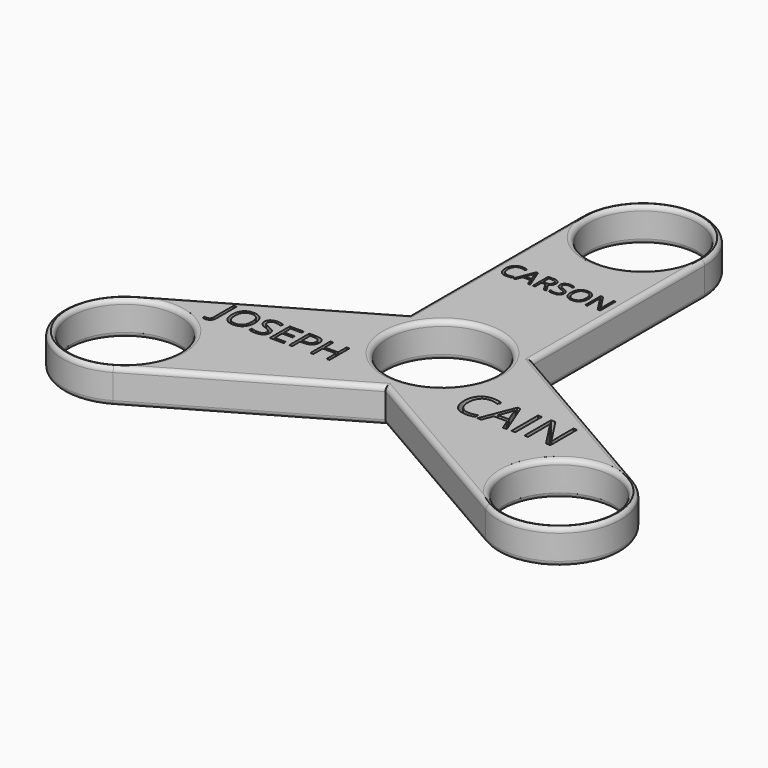
from build123d import *

# Parameters (mm, degrees)
F2_DEPTH      = 7
F1_R          = 11
F1_R_2        = 11.1
F3_DEPTH      = 25.4
F4_T8_DEPTH   = 46.0831216351
F4_T13_DEPTH  = 46.0831216351
F4_T18_DEPTH  = 46.0831216351
F4_T23_DEPTH  = 46.0831216351
F4_T28_DEPTH  = 46.0831216351
F4_T37_DEPTH  = 46.0831216351
F4_T42_DEPTH  = 46.0831216351
F4_T51_DEPTH  = 46.0831216351
F4_T56_DEPTH  = 46.0831216351
F4_T59_ANGLE  = 180
F4_T61_ANGLE  = 180
F4_T63_ANGLE  = 180
F4_T67_DEPTH  = 46.0831216351
F4_T70_ANGLE  = 180
F4_T74_DEPTH  = 46.0831216351
F4_T77_ANGLE  = 180
F4_T81_DEPTH  = 46.0831216351
F4_T84_ANGLE  = 180
F4_T89_DEPTH  = 46.0831216351
F4_T93_DEPTH  = 46.0831216351
F4_T100_DEPTH = 46.0831216351
F4_T104_DEPTH = 46.0831216351
F4_T111_DEPTH = 46.0831216351
F4_T115_DEPTH = 46.0831216351
F4_T122_DEPTH = 46.0831216351
F4_T126_DEPTH = 46.0831216351
F4_T133_DEPTH = 46.0831216351
F4_T137_DEPTH = 46.0831216351
F4_T144_DEPTH = 46.0831216351
F4_T148_DEPTH = 46.0831216351
F5_R          = 1
F6_TEXT_SIZE  = 5.4523334279
F7_DEPTH      = 3
F8_TEXT_SIZE  = 7.1097765769
F9_DEPTH      = 3
F10_TEXT_SIZE = 9.4424461066
F11_DEPTH     = 3


# Not quite as in the source:
# - a fillet or chamfer that OpenCascade refuses, or shapes differently, is made with other operations: its cross-section is extruded or revolved along the edge and cut away or added
# - Text() gives the source's letters only with a copy of the font that has no kerning and outlines rounded to 1/6400 em; it was checked with that copy


with BuildPart() as f2:
    # F0 (on Top) → F2 (new body)
    with BuildSketch(Plane.XY):
        with BuildLine():
            ThreePointArc((12.5, 50.8), (0, 63.3), (-12.5, 50.8))
            Line((-12.5, 50.8), (-12.5, 7.2168783649))
            Line((-12.5, 7.2168783649), (-50.2440905122, -14.5746824527))
            ThreePointArc((-50.2440905122, -14.5746824527), (-54.8194080596, -31.65), (-37.7440905122, -36.2253175473))
            Line((-37.7440905122, -36.2253175473), (0, -14.4337567297))
            Line((0, -14.4337567297), (37.7440905122, -36.2253175473))
            ThreePointArc((37.7440905122, -36.2253175473), (54.8194080596, -31.65), (50.2440905122, -14.5746824527))
            Line((50.2440905122, -14.5746824527), (12.5, 7.2168783649))
            Line((12.5, 7.2168783649), (12.5, 50.8))
        make_face()
    extrude(amount=F2_DEPTH)

    # F1 (on Top) → F3 (cut)
    with BuildSketch(Plane.XY):
        with Locations((0, 50.8)):
            Circle(F1_R)
        with Locations((-43.9940905122, -25.4)):
            Circle(F1_R)
        with Locations((43.9940905122, -25.4)):
            Circle(F1_R)
        Circle(F1_R_2)
    extrude(amount=F3_DEPTH, mode=Mode.SUBTRACT)

    # F4: fillet of radius 1 on 15 edges, made by hand

    # F4_s1 → F4_t2 (revolve, cut)
    with BuildSketch(Plane.XZ.offset(-50.8)):
        with BuildLine():
            ThreePointArc((12, 7), (11.2928932188, 6.7071067812), (11, 6))
            Line((11, 6), (11, 7))
            Line((11, 7), (12, 7))
        make_face()
    revolve(axis=Axis((0, 50.8, 7), (0, 0, -1)), mode=Mode.SUBTRACT)

    # F4_s3 → F4_t4 (revolve, cut)
    with BuildSketch(Plane.XZ.offset(-50.8)):
        with BuildLine():
            ThreePointArc((12, 0), (11.2928932188, 0.2928932188), (11, 1))
            Line((11, 1), (11, 0))
            Line((11, 0), (12, 0))
        make_face()
    revolve(axis=Axis((0, 50.8, 0), (0, 0, 1)), mode=Mode.SUBTRACT)


with BuildPart() as f4_tool6:
    # F4_s7 → F4_t8 (new body)
    with BuildSketch(Plane.XZ.offset(-50.8)):
        with BuildLine():
            ThreePointArc((-11.5, 0), (-12.2071067812, 0.2928932188), (-12.5, 1))
            Line((-12.5, 1), (-12.5, 0))
            Line((-12.5, 0), (-11.5, 0))
        make_face()
    extrude(amount=F4_T8_DEPTH)

    split(bisect_by=Plane(origin=(-6.25, 10.8253175473, 0), x_dir=(0, 0, 1), z_dir=(-0.5, 0.8660254038, 0)), keep=Keep.TOP)


with BuildPart() as f2_1:
    add(f2.part)

    # F4_t5: cut F4_tool6
    add(f4_tool6.part, mode=Mode.SUBTRACT)


with BuildPart() as f4_tool11:
    # F4_s12 → F4_t13 (new body)
    with BuildSketch(Plane.XZ.offset(-4.7168783649)):
        with BuildLine():
            ThreePointArc((11.5, 0), (12.2071067812, 0.2928932188), (12.5, 1))
            Line((12.5, 1), (12.5, 0))
            Line((12.5, 0), (11.5, 0))
        make_face()
    extrude(amount=-F4_T13_DEPTH)

    split(bisect_by=Plane(origin=(6.25, 10.8253175473, 0), x_dir=(0, 0, 1), z_dir=(0.5, 0.8660254038, 0)), keep=Keep.TOP)


with BuildPart() as f2_2:
    add(f2_1.part)

    # F4_t10: cut F4_tool11
    add(f4_tool11.part, mode=Mode.SUBTRACT)


with BuildPart() as f4_tool16:
    # F4_s17 → F4_t18 (new body)
    with BuildSketch(Plane.XZ.offset(-4.7168783649)):
        with BuildLine():
            ThreePointArc((11.5, 7), (12.2071067812, 6.7071067812), (12.5, 6))
            Line((12.5, 6), (12.5, 7))
            Line((12.5, 7), (11.5, 7))
        make_face()
    extrude(amount=-F4_T18_DEPTH)

    split(bisect_by=Plane(origin=(6.25, 10.8253175473, 0), x_dir=(0, 0, 1), z_dir=(0.5, 0.8660254038, 0)), keep=Keep.TOP)


with BuildPart() as f2_3:
    add(f2_2.part)

    # F4_t15: cut F4_tool16
    add(f4_tool16.part, mode=Mode.SUBTRACT)


with BuildPart() as f4_tool21:
    # F4_s22 → F4_t23 (new body)
    with BuildSketch(Plane(origin=(-4.0849364905, -2.3584391824, 0), x_dir=(0, 0, 1), z_dir=(-0.8660254038, -0.5, 0))):
        with BuildLine():
            ThreePointArc((0, 11.5), (0.2928932188, 12.2071067812), (1, 12.5))
            Line((1, 12.5), (0, 12.5))
            Line((0, 12.5), (0, 11.5))
        make_face()
    extrude(amount=F4_T23_DEPTH)

    split(bisect_by=Plane.YZ.offset(-12.5), keep=Keep.BOTTOM)


with BuildPart() as f2_4:
    add(f2_3.part)

    # F4_t20: cut F4_tool21
    add(f4_tool21.part, mode=Mode.SUBTRACT)


with BuildPart() as f4_tool26:
    # F4_s27 → F4_t28 (new body)
    with BuildSketch(Plane(origin=(-4.0849364905, -2.3584391824, 0), x_dir=(0, 0, 1), z_dir=(-0.8660254038, -0.5, 0))):
        with BuildLine():
            ThreePointArc((7, 11.5), (6.7071067812, 12.2071067812), (6, 12.5))
            Line((6, 12.5), (7, 12.5))
            Line((7, 12.5), (7, 11.5))
        make_face()
    extrude(amount=F4_T28_DEPTH)

    split(bisect_by=Plane.YZ.offset(-12.5), keep=Keep.BOTTOM)


with BuildPart() as f2_5:
    add(f2_4.part)

    # F4_t25: cut F4_tool26
    add(f4_tool26.part, mode=Mode.SUBTRACT)

    # F4_s30 → F4_t31 (revolve, cut)
    with BuildSketch(Plane.XZ.offset(25.4)):
        with BuildLine():
            ThreePointArc((-31.9940905122, 0), (-32.7011972934, 0.2928932188), (-32.9940905122, 1))
            Line((-32.9940905122, 1), (-32.9940905122, 0))
            Line((-32.9940905122, 0), (-31.9940905122, 0))
        make_face()
    revolve(axis=Axis((-43.9940905122, -25.4, 0), (0, 0, 1)), mode=Mode.SUBTRACT)

    # F4_s32 → F4_t33 (revolve, cut)
    with BuildSketch(Plane.XZ.offset(25.4)):
        with BuildLine():
            ThreePointArc((-31.9940905122, 7), (-32.7011972934, 6.7071067812), (-32.9940905122, 6))
            Line((-32.9940905122, 6), (-32.9940905122, 7))
            Line((-32.9940905122, 7), (-31.9940905122, 7))
        make_face()
    revolve(axis=Axis((-43.9940905122, -25.4, 7), (0, 0, -1)), mode=Mode.SUBTRACT)


with BuildPart() as f4_tool35:
    # F4_s36 → F4_t37 (new body)
    with BuildSketch(Plane(origin=(43.9940905122, -25.4, 0), x_dir=(0, 0, 1), z_dir=(-0.8660254038, 0.5, 0))):
        with BuildLine():
            ThreePointArc((7, 11.5), (6.7071067812, 12.2071067812), (6, 12.5))
            Line((6, 12.5), (7, 12.5))
            Line((7, 12.5), (7, 11.5))
        make_face()
    extrude(amount=F4_T37_DEPTH)

    split(bisect_by=Plane.YZ.offset(12.5), keep=Keep.TOP)


with BuildPart() as f2_6:
    add(f2_5.part)

    # F4_t34: cut F4_tool35
    add(f4_tool35.part, mode=Mode.SUBTRACT)


with BuildPart() as f4_tool40:
    # F4_s41 → F4_t42 (new body)
    with BuildSketch(Plane(origin=(4.0849364905, -2.3584391824, 0), x_dir=(0, 0, 1), z_dir=(0.8660254038, -0.5, 0))):
        with BuildLine():
            ThreePointArc((6, 12.5), (6.7071067812, 12.2071067812), (7, 11.5))
            Line((7, 11.5), (7, 12.5))
            Line((7, 12.5), (6, 12.5))
        make_face()
    extrude(amount=F4_T42_DEPTH)

    split(bisect_by=Plane(origin=(6.25, -10.8253175473, 0), x_dir=(0, 0, 1), z_dir=(0.5, -0.8660254038, 0)), keep=Keep.TOP)


with BuildPart() as f2_7:
    add(f2_6.part)

    # F4_t39: cut F4_tool40
    add(f4_tool40.part, mode=Mode.SUBTRACT)

    # F4_s44 → F4_t45 (revolve, cut)
    with BuildSketch(Plane.XZ.offset(25.4)):
        with BuildLine():
            ThreePointArc((55.9940905122, 7), (55.2869837311, 6.7071067812), (54.9940905122, 6))
            Line((54.9940905122, 6), (54.9940905122, 7))
            Line((54.9940905122, 7), (55.9940905122, 7))
        make_face()
    revolve(axis=Axis((43.9940905122, -25.4, 7), (0, 0, -1)), mode=Mode.SUBTRACT)

    # F4_s46 → F4_t47 (revolve, cut)
    with BuildSketch(Plane.XZ.offset(25.4)):
        with BuildLine():
            ThreePointArc((55.9940905122, 0), (55.2869837311, 0.2928932188), (54.9940905122, 1))
            Line((54.9940905122, 1), (54.9940905122, 0))
            Line((54.9940905122, 0), (55.9940905122, 0))
        make_face()
    revolve(axis=Axis((43.9940905122, -25.4, 0), (0, 0, 1)), mode=Mode.SUBTRACT)


with BuildPart() as f4_tool49:
    # F4_s50 → F4_t51 (new body)
    with BuildSketch(Plane(origin=(4.0849364905, -2.3584391824, 0), x_dir=(0, 0, 1), z_dir=(0.8660254038, -0.5, 0))):
        with BuildLine():
            ThreePointArc((1, 12.5), (0.2928932188, 12.2071067812), (0, 11.5))
            Line((0, 11.5), (0, 12.5))
            Line((0, 12.5), (1, 12.5))
        make_face()
    extrude(amount=F4_T51_DEPTH)

    split(bisect_by=Plane(origin=(6.25, -10.8253175473, 0), x_dir=(0, 0, 1), z_dir=(0.5, -0.8660254038, 0)), keep=Keep.TOP)


with BuildPart() as f2_8:
    add(f2_7.part)

    # F4_t48: cut F4_tool49
    add(f4_tool49.part, mode=Mode.SUBTRACT)


with BuildPart() as f4_tool54:
    # F4_s55 → F4_t56 (new body)
    with BuildSketch(Plane(origin=(43.9940905122, -25.4, 0), x_dir=(0, 0, 1), z_dir=(-0.8660254038, 0.5, 0))):
        with BuildLine():
            ThreePointArc((0, 11.5), (0.2928932188, 12.2071067812), (1, 12.5))
            Line((1, 12.5), (0, 12.5))
            Line((0, 12.5), (0, 11.5))
        make_face()
    extrude(amount=F4_T56_DEPTH)

    split(bisect_by=Plane.YZ.offset(12.5), keep=Keep.TOP)


with BuildPart() as f2_9:
    add(f2_8.part)

    # F4_t53: cut F4_tool54
    add(f4_tool54.part, mode=Mode.SUBTRACT)

    # F4_s58 → F4_t59 (revolve, cut)
    with BuildSketch(Plane(origin=(43.9940905122, -25.4, 0), x_dir=(0, 0, 1), z_dir=(-0.8660254038, 0.5, 0))):
        with BuildLine():
            ThreePointArc((0, -11.5), (0.2928932188, -12.2071067812), (1, -12.5))
            Line((1, -12.5), (0, -12.5))
            Line((0, -12.5), (0, -11.5))
        make_face()
    revolve(axis=Axis((43.9940905122, -25.4, 0), (0, 0, 1)), revolution_arc=F4_T59_ANGLE, mode=Mode.SUBTRACT)

    # F4_s60 → F4_t61 (revolve, cut)
    with BuildSketch(Plane(origin=(43.9940905122, -25.4, 0), x_dir=(0, 0, 1), z_dir=(-0.8660254038, 0.5, 0))):
        with BuildLine():
            ThreePointArc((7, -11.5), (6.7071067812, -12.2071067812), (6, -12.5))
            Line((6, -12.5), (7, -12.5))
            Line((7, -12.5), (7, -11.5))
        make_face()
    revolve(axis=Axis((43.9940905122, -25.4, 7), (0, 0, 1)), revolution_arc=F4_T61_ANGLE, mode=Mode.SUBTRACT)

    # F4_s62 → F4_t63 (revolve, cut)
    with BuildSketch(Plane(origin=(-43.9940905122, -25.4, 0), x_dir=(0, 0, 1), z_dir=(0.8660254038, 0.5, 0))):
        with BuildLine():
            ThreePointArc((6, -12.5), (6.7071067812, -12.2071067812), (7, -11.5))
            Line((7, -11.5), (7, -12.5))
            Line((7, -12.5), (6, -12.5))
        make_face()
    revolve(axis=Axis((-43.9940905122, -25.4, 7), (0, 0, 1)), revolution_arc=F4_T63_ANGLE, mode=Mode.SUBTRACT)


with BuildPart() as f4_tool65:
    # F4_s66 → F4_t67 (new body)
    with BuildSketch(Plane(origin=(-43.9940905122, -25.4, 0), x_dir=(0, 0, 1), z_dir=(0.8660254038, 0.5, 0))):
        with BuildLine():
            ThreePointArc((6, 12.5), (6.7071067812, 12.2071067812), (7, 11.5))
            Line((7, 11.5), (7, 12.5))
            Line((7, 12.5), (6, 12.5))
        make_face()
    extrude(amount=F4_T67_DEPTH)

    split(bisect_by=Plane(origin=(-6.25, -10.8253175473, 0), x_dir=(0, 0, 1), z_dir=(-0.5, -0.8660254038, 0)), keep=Keep.TOP)


with BuildPart() as f2_10:
    add(f2_9.part)

    # F4_t64: cut F4_tool65
    add(f4_tool65.part, mode=Mode.SUBTRACT)

    # F4_s69 → F4_t70 (revolve, cut)
    with BuildSketch(Plane(origin=(-43.9940905122, -25.4, 0), x_dir=(0, 0, 1), z_dir=(0.8660254038, 0.5, 0))):
        with BuildLine():
            ThreePointArc((1, -12.5), (0.2928932188, -12.2071067812), (0, -11.5))
            Line((0, -11.5), (0, -12.5))
            Line((0, -12.5), (1, -12.5))
        make_face()
    revolve(axis=Axis((-43.9940905122, -25.4, 0), (0, 0, 1)), revolution_arc=F4_T70_ANGLE, mode=Mode.SUBTRACT)


with BuildPart() as f4_tool72:
    # F4_s73 → F4_t74 (new body)
    with BuildSketch(Plane(origin=(-43.9940905122, -25.4, 0), x_dir=(0, 0, 1), z_dir=(0.8660254038, 0.5, 0))):
        with BuildLine():
            ThreePointArc((1, 12.5), (0.2928932188, 12.2071067812), (0, 11.5))
            Line((0, 11.5), (0, 12.5))
            Line((0, 12.5), (1, 12.5))
        make_face()
    extrude(amount=F4_T74_DEPTH)

    split(bisect_by=Plane(origin=(-6.25, -10.8253175473, 0), x_dir=(0, 0, 1), z_dir=(-0.5, -0.8660254038, 0)), keep=Keep.TOP)


with BuildPart() as f2_11:
    add(f2_10.part)

    # F4_t71: cut F4_tool72
    add(f4_tool72.part, mode=Mode.SUBTRACT)

    # F4_s76 → F4_t77 (revolve, cut)
    with BuildSketch(Plane.XZ.offset(-50.8)):
        with BuildLine():
            ThreePointArc((11.5, 7), (12.2071067812, 6.7071067812), (12.5, 6))
            Line((12.5, 6), (12.5, 7))
            Line((12.5, 7), (11.5, 7))
        make_face()
    revolve(axis=Axis((0, 50.8, 7), (0, 0, 1)), revolution_arc=F4_T77_ANGLE, mode=Mode.SUBTRACT)


with BuildPart() as f4_tool79:
    # F4_s80 → F4_t81 (new body)
    with BuildSketch(Plane.XZ.offset(-50.8)):
        with BuildLine():
            ThreePointArc((-11.5, 7), (-12.2071067812, 6.7071067812), (-12.5, 6))
            Line((-12.5, 6), (-12.5, 7))
            Line((-12.5, 7), (-11.5, 7))
        make_face()
    extrude(amount=F4_T81_DEPTH)

    split(bisect_by=Plane(origin=(-6.25, 10.8253175473, 0), x_dir=(0, 0, 1), z_dir=(-0.5, 0.8660254038, 0)), keep=Keep.TOP)


with BuildPart() as f2_12:
    add(f2_11.part)

    # F4_t78: cut F4_tool79
    add(f4_tool79.part, mode=Mode.SUBTRACT)

    # F4_s83 → F4_t84 (revolve, cut)
    with BuildSketch(Plane.XZ.offset(-50.8)):
        with BuildLine():
            ThreePointArc((11.5, 0), (12.2071067812, 0.2928932188), (12.5, 1))
            Line((12.5, 1), (12.5, 0))
            Line((12.5, 0), (11.5, 0))
        make_face()
    revolve(axis=Axis((0, 50.8, 0), (0, 0, 1)), revolution_arc=F4_T84_ANGLE, mode=Mode.SUBTRACT)


with BuildPart() as f4_tool87:
    # F4_s88 → F4_t89 (new body)
    with BuildSketch(Plane(origin=(-4.0849364905, -2.3584391824, 0), x_dir=(0, 0, 1), z_dir=(-0.8660254038, -0.5, 0))):
        with BuildLine():
            ThreePointArc((0, 11.5), (0.2928932188, 12.2071067812), (1, 12.5))
            Line((1, 12.5), (0, 12.5))
            Line((0, 12.5), (0, 11.5))
        make_face()
    extrude(amount=F4_T89_DEPTH)

    split(bisect_by=Plane.YZ.offset(-12.5), keep=Keep.TOP)


with BuildPart() as f4_tool91:
    # F4_s92 → F4_t93 (new body)
    with BuildSketch(Plane.XZ.offset(-50.8)):
        with BuildLine():
            ThreePointArc((-11.5, 0), (-12.2071067812, 0.2928932188), (-12.5, 1))
            Line((-12.5, 1), (-12.5, 0))
            Line((-12.5, 0), (-11.5, 0))
        make_face()
    extrude(amount=F4_T93_DEPTH)

    split(bisect_by=Plane(origin=(-6.25, 10.8253175473, 0), x_dir=(0, 0, 1), z_dir=(0.5, -0.8660254038, 0)), keep=Keep.TOP)


with BuildPart() as f4_tool87_1:
    add(f4_tool87.part)

    # F4_t95: intersect F4_tool91
    add(f4_tool91.part, mode=Mode.INTERSECT)


with BuildPart() as f2_13:
    add(f2_12.part)

    # F4_t85: cut F4_tool87
    add(f4_tool87_1.part, mode=Mode.SUBTRACT)


with BuildPart() as f4_tool98:
    # F4_s99 → F4_t100 (new body)
    with BuildSketch(Plane(origin=(43.9940905122, -25.4, 0), x_dir=(0, 0, 1), z_dir=(-0.8660254038, 0.5, 0))):
        with BuildLine():
            ThreePointArc((0, 11.5), (0.2928932188, 12.2071067812), (1, 12.5))
            Line((1, 12.5), (0, 12.5))
            Line((0, 12.5), (0, 11.5))
        make_face()
    extrude(amount=F4_T100_DEPTH)

    split(bisect_by=Plane.YZ.offset(12.5), keep=Keep.BOTTOM)


with BuildPart() as f4_tool102:
    # F4_s103 → F4_t104 (new body)
    with BuildSketch(Plane.XZ.offset(-4.7168783649)):
        with BuildLine():
            ThreePointArc((11.5, 0), (12.2071067812, 0.2928932188), (12.5, 1))
            Line((12.5, 1), (12.5, 0))
            Line((12.5, 0), (11.5, 0))
        make_face()
    extrude(amount=-F4_T104_DEPTH)

    split(bisect_by=Plane(origin=(6.25, 10.8253175473, 0), x_dir=(0, 0, 1), z_dir=(-0.5, -0.8660254038, 0)), keep=Keep.TOP)


with BuildPart() as f4_tool98_1:
    add(f4_tool98.part)

    # F4_t106: intersect F4_tool102
    add(f4_tool102.part, mode=Mode.INTERSECT)


with BuildPart() as f2_14:
    add(f2_13.part)

    # F4_t96: cut F4_tool98
    add(f4_tool98_1.part, mode=Mode.SUBTRACT)


with BuildPart() as f4_tool109:
    # F4_s110 → F4_t111 (new body)
    with BuildSketch(Plane(origin=(43.9940905122, -25.4, 0), x_dir=(0, 0, 1), z_dir=(-0.8660254038, 0.5, 0))):
        with BuildLine():
            ThreePointArc((7, 11.5), (6.7071067812, 12.2071067812), (6, 12.5))
            Line((6, 12.5), (7, 12.5))
            Line((7, 12.5), (7, 11.5))
        make_face()
    extrude(amount=F4_T111_DEPTH)

    split(bisect_by=Plane.YZ.offset(12.5), keep=Keep.BOTTOM)


with BuildPart() as f4_tool113:
    # F4_s114 → F4_t115 (new body)
    with BuildSketch(Plane.XZ.offset(-4.7168783649)):
        with BuildLine():
            ThreePointArc((11.5, 7), (12.2071067812, 6.7071067812), (12.5, 6))
            Line((12.5, 6), (12.5, 7))
            Line((12.5, 7), (11.5, 7))
        make_face()
    extrude(amount=-F4_T115_DEPTH)

    split(bisect_by=Plane(origin=(6.25, 10.8253175473, 0), x_dir=(0, 0, 1), z_dir=(-0.5, -0.8660254038, 0)), keep=Keep.TOP)


with BuildPart() as f4_tool109_1:
    add(f4_tool109.part)

    # F4_t117: intersect F4_tool113
    add(f4_tool113.part, mode=Mode.INTERSECT)


with BuildPart() as f2_15:
    add(f2_14.part)

    # F4_t107: cut F4_tool109
    add(f4_tool109_1.part, mode=Mode.SUBTRACT)


with BuildPart() as f4_tool120:
    # F4_s121 → F4_t122 (new body)
    with BuildSketch(Plane(origin=(-4.0849364905, -2.3584391824, 0), x_dir=(0, 0, 1), z_dir=(-0.8660254038, -0.5, 0))):
        with BuildLine():
            ThreePointArc((7, 11.5), (6.7071067812, 12.2071067812), (6, 12.5))
            Line((6, 12.5), (7, 12.5))
            Line((7, 12.5), (7, 11.5))
        make_face()
    extrude(amount=F4_T122_DEPTH)

    split(bisect_by=Plane.YZ.offset(-12.5), keep=Keep.TOP)


with BuildPart() as f4_tool124:
    # F4_s125 → F4_t126 (new body)
    with BuildSketch(Plane.XZ.offset(-50.8)):
        with BuildLine():
            ThreePointArc((-11.5, 7), (-12.2071067812, 6.7071067812), (-12.5, 6))
            Line((-12.5, 6), (-12.5, 7))
            Line((-12.5, 7), (-11.5, 7))
        make_face()
    extrude(amount=F4_T126_DEPTH)

    split(bisect_by=Plane(origin=(-6.25, 10.8253175473, 0), x_dir=(0, 0, 1), z_dir=(0.5, -0.8660254038, 0)), keep=Keep.TOP)


with BuildPart() as f4_tool120_1:
    add(f4_tool120.part)

    # F4_t128: intersect F4_tool124
    add(f4_tool124.part, mode=Mode.INTERSECT)


with BuildPart() as f2_16:
    add(f2_15.part)

    # F4_t118: cut F4_tool120
    add(f4_tool120_1.part, mode=Mode.SUBTRACT)


with BuildPart() as f4_tool131:
    # F4_s132 → F4_t133 (new body)
    with BuildSketch(Plane(origin=(-43.9940905122, -25.4, 0), x_dir=(0, 0, 1), z_dir=(0.8660254038, 0.5, 0))):
        with BuildLine():
            ThreePointArc((6, 12.5), (6.7071067812, 12.2071067812), (7, 11.5))
            Line((7, 11.5), (7, 12.5))
            Line((7, 12.5), (6, 12.5))
        make_face()
    extrude(amount=F4_T133_DEPTH)

    split(bisect_by=Plane(origin=(-6.25, -10.8253175473, 0), x_dir=(0, 0, 1), z_dir=(0.5, 0.8660254038, 0)), keep=Keep.TOP)


with BuildPart() as f4_tool135:
    # F4_s136 → F4_t137 (new body)
    with BuildSketch(Plane(origin=(4.0849364905, -2.3584391824, 0), x_dir=(0, 0, 1), z_dir=(0.8660254038, -0.5, 0))):
        with BuildLine():
            ThreePointArc((6, 12.5), (6.7071067812, 12.2071067812), (7, 11.5))
            Line((7, 11.5), (7, 12.5))
            Line((7, 12.5), (6, 12.5))
        make_face()
    extrude(amount=F4_T137_DEPTH)

    split(bisect_by=Plane(origin=(6.25, -10.8253175473, 0), x_dir=(0, 0, 1), z_dir=(-0.5, 0.8660254038, 0)), keep=Keep.TOP)


with BuildPart() as f4_tool131_1:
    add(f4_tool131.part)

    # F4_t139: intersect F4_tool135
    add(f4_tool135.part, mode=Mode.INTERSECT)


with BuildPart() as f2_17:
    add(f2_16.part)

    # F4_t129: cut F4_tool131
    add(f4_tool131_1.part, mode=Mode.SUBTRACT)


with BuildPart() as f4_tool142:
    # F4_s143 → F4_t144 (new body)
    with BuildSketch(Plane(origin=(-43.9940905122, -25.4, 0), x_dir=(0, 0, 1), z_dir=(0.8660254038, 0.5, 0))):
        with BuildLine():
            ThreePointArc((1, 12.5), (0.2928932188, 12.2071067812), (0, 11.5))
            Line((0, 11.5), (0, 12.5))
            Line((0, 12.5), (1, 12.5))
        make_face()
    extrude(amount=F4_T144_DEPTH)

    split(bisect_by=Plane(origin=(-6.25, -10.8253175473, 0), x_dir=(0, 0, 1), z_dir=(0.5, 0.8660254038, 0)), keep=Keep.TOP)


with BuildPart() as f4_tool146:
    # F4_s147 → F4_t148 (new body)
    with BuildSketch(Plane(origin=(4.0849364905, -2.3584391824, 0), x_dir=(0, 0, 1), z_dir=(0.8660254038, -0.5, 0))):
        with BuildLine():
            ThreePointArc((1, 12.5), (0.2928932188, 12.2071067812), (0, 11.5))
            Line((0, 11.5), (0, 12.5))
            Line((0, 12.5), (1, 12.5))
        make_face()
    extrude(amount=F4_T148_DEPTH)

    split(bisect_by=Plane(origin=(6.25, -10.8253175473, 0), x_dir=(0, 0, 1), z_dir=(-0.5, 0.8660254038, 0)), keep=Keep.TOP)


with BuildPart() as f4_tool142_1:
    add(f4_tool142.part)

    # F4_t150: intersect F4_tool146
    add(f4_tool146.part, mode=Mode.INTERSECT)


with BuildPart() as f2_18:
    add(f2_17.part)

    # F4_t140: cut F4_tool142
    add(f4_tool142_1.part, mode=Mode.SUBTRACT)

    # F5
    f5_edges = [f2_18.edges().sort_by_distance(p)[0] for p in [
        (-11.1, 0, 7),
        (-11.1, 0, 0),
    ]]
    fillet(f5_edges, radius=F5_R)

    # F6 (on face) → F7 (cut)
    with BuildSketch(Plane.XY.offset(7)):
        with Locations((-10.7142611494, 27.0058503977)):
            Text('CARSON', F6_TEXT_SIZE, font='Open Sans', text_align=(TextAlign.LEFT, TextAlign.BOTTOM))
    extrude(amount=-F7_DEPTH, mode=Mode.SUBTRACT)

    # F8 (on face) → F9 (cut)
    with BuildSketch(Plane.XY.offset(7)):
        with Locations((-36.6326735651, -12.9898668879)):
            Text('JOSEPH', F8_TEXT_SIZE, font='Open Sans', text_align=(TextAlign.LEFT, TextAlign.BOTTOM))
    extrude(amount=-F9_DEPTH, mode=Mode.SUBTRACT)

    # F10 (on face) → F11 (cut)
    with BuildSketch(Plane.XY.offset(7)):
        with Locations((12.2769270092, -13.9505891129)):
            Text('CAIN', F10_TEXT_SIZE, font='Open Sans', text_align=(TextAlign.LEFT, TextAlign.BOTTOM))
    extrude(amount=-F11_DEPTH, mode=Mode.SUBTRACT)


solid = f2_18.part
